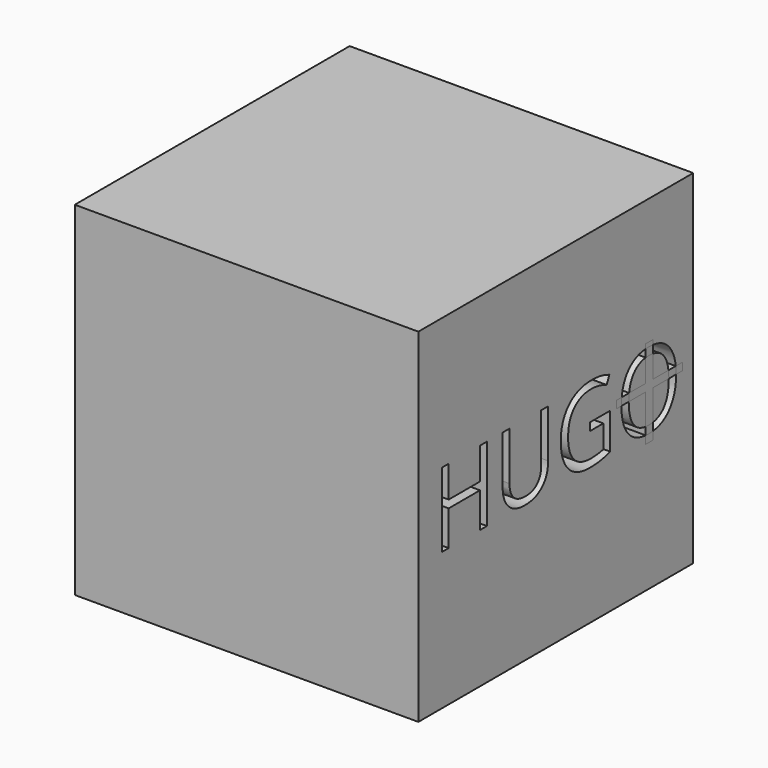
from build123d import *

# Parameters (mm, degrees)
F0_W         = 55
F0_H         = 55
F1_DEPTH     = 55
F2_TEXT_SIZE = 16.6666666667
F3_DEPTH     = 55.001
F4_W         = 5.8199428022
F4_H         = 1.2003914836
F4_W_2       = 1.4467900619
F4_H_2       = 7.3805688497
F4_W_3       = 5.8869377244
F4_H_3       = 5.5876020342
F5_DEPTH     = 55


# Not quite as in the source:
# - Text() gives the source's letters only with a copy of the font that has no kerning and outlines rounded to 1/6400 em; it was checked with that copy


with BuildPart() as f1:
    # F0 (on Right) → F1 (new body)
    with BuildSketch(Plane.YZ):
        with Locations((-27.5, 27.5)):
            Rectangle(F0_W, F0_H)
    extrude(amount=F1_DEPTH)

    # F2 (on face) → F3 (cut, through all)
    with BuildSketch(Plane.YZ.offset(55)):
        with Locations((-51.9469958063, 22.0296363658)):
            Text('HUGO', F2_TEXT_SIZE, font='Open Sans', text_align=(TextAlign.LEFT, TextAlign.BOTTOM))
    extrude(amount=-F3_DEPTH, mode=Mode.SUBTRACT)

    # F4 (on face) → F5 (join, through all)
    with BuildSketch(Plane(origin=(0, 0, 0), x_dir=(0, -1, 0), z_dir=(-1, 0, 0))):
        with Locations((12.4116260558, 28.611602941)):
            Rectangle(F4_W, F4_H)
        with Locations((8.7782596238, 24.3211227743)):
            Rectangle(F4_W_2, F4_H_2)
        with Locations((8.7782596238, 28.611602941)):
            Rectangle(F4_W_2, F4_H)
        with Locations((5.1113957306, 28.611602941)):
            Rectangle(F4_W_3, F4_H)
        with Locations((8.7782596238, 32.0055996999)):
            Rectangle(F4_W_2, F4_H_3)
    extrude(amount=-F5_DEPTH)


solid = f1.part
